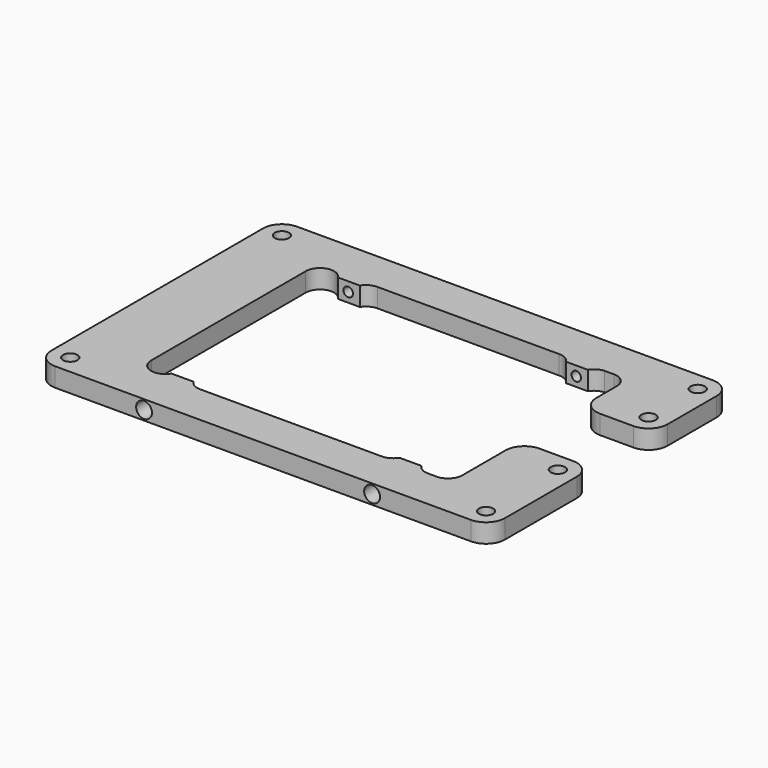
from build123d import *

# Parameters (mm, degrees)
F0_R           = 2.413
F1_DEPTH       = 6.35
F3_D           = 3.175
F3_DEPTH       = 15.875
F3_CBORE_D     = 5.334
F3_CBORE_DEPTH = 6.35
F3_TIP         = 0.9538662327
F5_D           = 3.175
F5_DEPTH       = 15.875
F5_CBORE_D     = 5.334
F5_CBORE_DEPTH = 6.35
F5_TIP         = 0.9538662327


# Not quite as in the source:
# - ends of sketch curves that miss each other by under 0.0002 mm in the source are joined


with BuildPart() as f1:
    # F0 (on Top) → F1 (new body)
    with BuildSketch(Plane.XY):
        with BuildLine():
            Line((69.85, 50.8), (-69.85, 50.8))
            ThreePointArc((-69.85, 50.8), (-74.3401280605, 48.9401280605), (-76.2, 44.45))
            Line((-76.2, 44.45), (-76.2, -44.45))
            ThreePointArc((-76.2, -44.45), (-74.3401280605, -48.9401280605), (-69.85, -50.8))
            Line((-69.85, -50.8), (69.85, -50.8))
            ThreePointArc((69.85, -50.8), (74.3401280605, -48.9401280605), (76.2, -44.45))
            Line((76.2, -44.45), (76.2, -14.2860641539))
            ThreePointArc((76.2, -14.2860641539), (74.3401280605, -9.7959360934), (69.85, -7.9360641539))
            Line((69.85, -7.9360641539), (58.6074946763, -7.9360641539))
            ThreePointArc((58.6074946763, -7.9360641539), (54.1173666157, -9.7959360934), (52.2574946763, -14.2860641539))
            Line((52.2574946763, -14.2860641539), (52.2574946763, -32.4625809134))
            ThreePointArc((52.2574946763, -32.4625809134), (50.8625907217, -35.8301769588), (47.4949946763, -37.2250809134))
            Line((47.4949946763, -37.2250809134), (44.3277485112, -37.2250809134))
            ThreePointArc((44.3277485112, -37.2250809134), (42.13331562, -36.5581056788), (40.5040542932, -34.9438258992))
            Line((40.5040542932, -34.9438258992), (33.1534721252, -34.9569741008))
            ThreePointArc((33.1534721252, -34.9569741008), (31.4174339307, -36.6267371458), (29.0867928871, -37.2350541396))
            Line((29.0867928871, -37.2350541396), (-32.0008653101, -37.2349356495))
            ThreePointArc((-32.0008653101, -37.2349356495), (-32.011823158, -37.2349229987), (-32.0227809478, -37.23488518))
            ThreePointArc((-32.0227809478, -37.23488518), (-34.343480333, -36.6189475252), (-36.0687477759, -34.9490741523))
            Line((-36.0687477759, -34.9490741523), (-43.4277583378, -34.9532397009))
            ThreePointArc((-43.4277583378, -34.9532397009), (-48.8402121166, -37.0437819519), (-52.2557695883, -32.3534738631))
            Line((-52.2557695883, -32.3534738631), (-52.2557695883, 32.3534738631))
            ThreePointArc((-52.2557695883, 32.3534738631), (-48.8402121166, 37.0437819519), (-43.4277583378, 34.9532397009))
            Line((-43.4277583378, 34.9532397009), (-36.0798295377, 34.9490804251))
            ThreePointArc((-36.0798295377, 34.9490804251), (-34.3499401325, 36.6220397206), (-32.0227811798, 37.2349356069))
            Line((-32.0227811798, 37.2349356069), (29.0868021404, 37.2350541396))
            ThreePointArc((29.0868021404, 37.2350541396), (31.4174339307, 36.6267371458), (33.1534721252, 34.9569741008))
            Line((33.1534721252, 34.9569741008), (40.5040542932, 34.9438258992))
            ThreePointArc((40.5040542932, 34.9438258992), (42.13331562, 36.5581056788), (44.3277485112, 37.2250809134))
            Line((44.3277485112, 37.2250809134), (47.4949946763, 37.2250809134))
            ThreePointArc((47.4949946763, 37.2250809134), (50.8625907217, 35.8301769588), (52.2574946763, 32.4625809134))
            Line((52.2574946763, 32.4625809134), (52.2574946763, 23.8139358461))
            ThreePointArc((52.2574946763, 23.8139358461), (54.1173666157, 19.3238077856), (58.6074946763, 17.4639358461))
            Line((58.6074946763, 17.4639358461), (69.85, 17.4639358461))
            ThreePointArc((69.85, 17.4639358461), (74.3401280605, 19.3238077856), (76.2, 23.8139358461))
            Line((76.2, 23.8139358461), (76.2, 44.45))
            ThreePointArc((76.2, 44.45), (74.3401280605, 48.9401280605), (69.85, 50.8))
        make_face()
        with Locations((-69.85, -44.45)):
            Circle(F0_R, mode=Mode.SUBTRACT)
        with Locations((69.85, -44.45)):
            Circle(F0_R, mode=Mode.SUBTRACT)
        with Locations((69.85, -14.2860641539)):
            Circle(F0_R, mode=Mode.SUBTRACT)
        with Locations((-69.85, 44.45)):
            Circle(F0_R, mode=Mode.SUBTRACT)
        with Locations((69.85, 23.8139358461)):
            Circle(F0_R, mode=Mode.SUBTRACT)
        with Locations((69.85, 44.45)):
            Circle(F0_R, mode=Mode.SUBTRACT)
    extrude(amount=F1_DEPTH)

    # F3
    with Locations(Plane.XZ.offset(50.8)):
        with Locations((-39.9796, 3.175), (36.6377, 3.175)):
            CounterBoreHole(F3_D / 2, F3_CBORE_D / 2, F3_CBORE_DEPTH, depth=F3_DEPTH)
            with Locations((0, 0, -(F3_DEPTH + F3_TIP / 2))):  # 118° drill point
                Cone(0, F3_D / 2, F3_TIP, mode=Mode.SUBTRACT)

    # F5
    with Locations(Plane(origin=(0, 50.8, 0), x_dir=(-1, 0, 0), z_dir=(0, 1, 0))):
        with Locations((-36.6268, 3.175), (39.9796, 3.175)):
            CounterBoreHole(F5_D / 2, F5_CBORE_D / 2, F5_CBORE_DEPTH, depth=F5_DEPTH)
            with Locations((0, 0, -(F5_DEPTH + F5_TIP / 2))):  # 118° drill point
                Cone(0, F5_D / 2, F5_TIP, mode=Mode.SUBTRACT)


solid = f1.part
